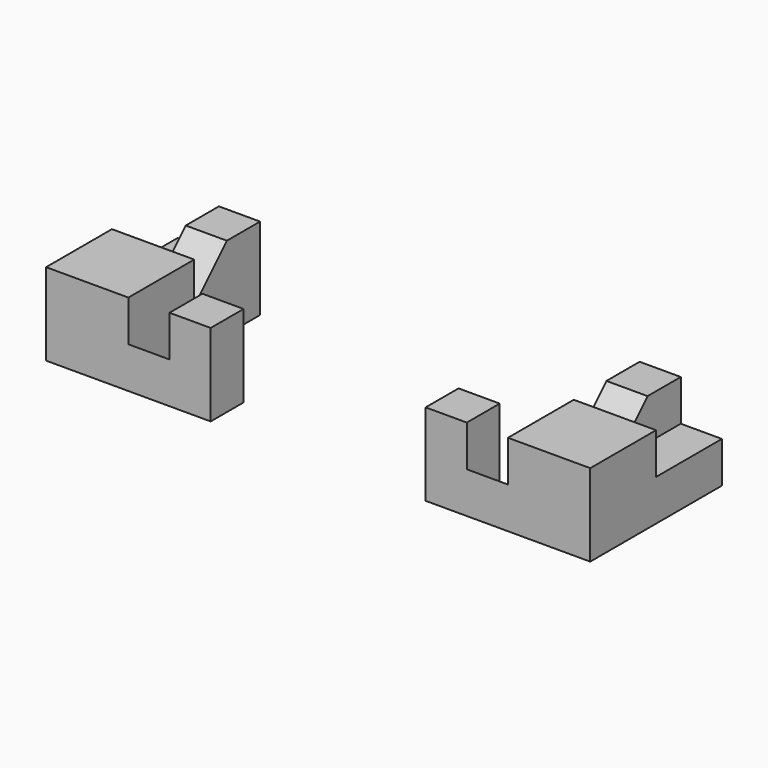
from build123d import *

# Parameters (mm, degrees)
F1_DEPTH  = 12.0904
F2_DEPTH  = 6.0452
F0_W      = 6.0452
F0_H      = 6.0452
F3_DEPTH  = 12.0904
F4_DEPTH  = 12.0904
F5_DEPTH  = 6.0452
F6_SIZE   = 6.04519
F7_DEPTH  = 12.0904
F8_DEPTH  = 12.0904
F11_DEPTH = 6.0452


# Not quite as in the source:
# - a fillet or chamfer is up to 0.001 mm smaller than in the source, because OpenCascade refuses the exact size


with BuildPart() as f1:
    # F0 (on Top) → F1 (new body)
    with BuildSketch(Plane.XY):
        Polygon((-39.9695653213, 0), (-27.8791653213, 0), (-27.8791653213, 6.0452), (-27.8791653213, 12.0904), (-33.9243653213, 12.0904), (-39.9695653213, 12.0904), align=None)
    extrude(amount=F1_DEPTH)

    # F0 (on Top) → F2 (join)
    with BuildSketch(Plane.XY):
        Polygon((-39.9695653213, 24.1808), (-39.9695653213, 12.0904), (-33.9243653213, 12.0904), (-33.9243653213, 18.1356), (-33.9243653213, 24.1808), align=None)
    extrude(amount=F2_DEPTH)

    # F0 (on Top) → F3 (join)
    with BuildSketch(Plane.XY):
        with Locations((-30.9017653213, 21.1582)):
            Rectangle(F0_W, F0_H)
    extrude(amount=F3_DEPTH)



with BuildPart() as f4:
    # F0 (on Top) → F4 (new body)
    with BuildSketch(Plane.XY):
        with Locations((-18.8113653213, 3.0226)):
            Rectangle(F0_W, F0_H)
    extrude(amount=F4_DEPTH)


with BuildPart() as f1_1:
    add(f1.part)

    add(f4.part)  # F5 merges F4
    # F0 (on Top) → F5 (join)
    with BuildSketch(Plane.XY):
        with Locations((-24.8565653213, 3.0226)):
            Rectangle(F0_W, F0_H)
    extrude(amount=F5_DEPTH)

    # F6 (size 6.0452 in the source; OpenCascade refuses exactly that, so slightly less here)
    f6_edges = [f1_1.edges().sort_by_distance(p)[0] for p in [
        (-24.856565, 6.0452, 6.0452),
    ]]
    chamfer(f6_edges, length=F6_SIZE)

    # F0 (on Top) → F7 (join)
    with BuildSketch(Plane.XY):
        with Locations((-18.8113653213, 3.0226)):
            Rectangle(F0_W, F0_H)
    extrude(amount=F7_DEPTH)

    # F0 (on Top) → F8 (join)
    with BuildSketch(Plane.XY):
        with Locations((-30.9017653213, 15.113)):
            Rectangle(F0_W, F0_H)
    extrude(amount=F8_DEPTH)

    # F10 (on face) → F11 (cut, through all)
    with BuildSketch(Plane(origin=(-33.9243653213, 0, 0), x_dir=(0, -1, 0), z_dir=(-1, 0, 0))):
        Polygon((-12.0904, 12.0904), (-18.0848, 12.0904), (-12.0904, 6.0452), align=None)
    extrude(amount=-F11_DEPTH, mode=Mode.SUBTRACT)


with BuildPart() as f12_1:
    # F12: instance of F1
    add(f1_1.part.mirror(Plane.YZ))


solid = Compound([f1_1.part, f12_1.part])
